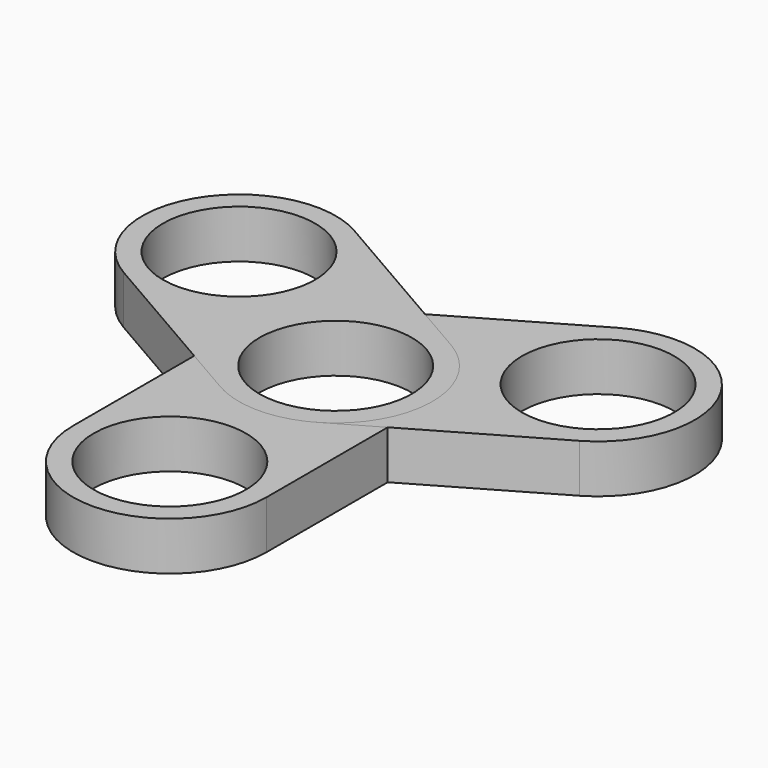
from build123d import *

# Parameters (mm, degrees)
F1_DEPTH        = 177.8
F1_COPIES_COUNT = 3


# Not quite as in the source:
# - a feature of the source that left no trace in its solid (it failed there, or was rolled back) is left out
# - a pattern or mirror of a feature is missing from the dataset's text; its kind, count and spacing are read off the source's solid


with BuildPart() as f1:
    # F0 (on Top) → F1 (new body)
    with BuildSketch(Plane.XY):
        with BuildLine():
            Line((711.2, 0), (635.635, 0))
            ThreePointArc((635.635, 0), (355.6, -280.035), (75.565, 0))
            Line((75.565, 0), (0, 0))
            ThreePointArc((0, 0), (355.6, -355.6), (711.2, 0))
        make_face()
        with BuildLine():
            ThreePointArc((75.565, 0), (355.6, 280.035), (635.635, 0))
            Line((635.635, 0), (711.2, 0))
            ThreePointArc((711.2, 0), (355.6, 355.6), (0, 0))
            Line((0, 0), (75.565, 0))
        make_face()
        with BuildLine():
            ThreePointArc((0, 0), (355.6, 355.6), (711.2, 0))
            Line((711.2, 0), (711.2, 762))
            ThreePointArc((711.2, 762), (355.6, 406.4), (0, 762))
            Line((0, 762), (0, 0))
        make_face()
        with BuildLine():
            Line((635.635, 762), (711.2, 762))
            ThreePointArc((711.2, 762), (355.6, 1117.6), (0, 762))
            Line((0, 762), (75.565, 762))
            ThreePointArc((75.565, 762), (355.6, 1042.035), (635.635, 762))
        make_face()
        with BuildLine():
            ThreePointArc((0, 762), (355.6, 406.4), (711.2, 762))
            Line((711.2, 762), (635.635, 762))
            ThreePointArc((635.635, 762), (355.6, 481.965), (75.565, 762))
            Line((75.565, 762), (0, 762))
        make_face()
    extrude(amount=F1_DEPTH)


with BuildPart() as f1_copies_1:
    # F1_copies: instance of F1
    add(f1.part.rotate(Axis((355.6, 762, 0), (0, 0, 1)), 1 * 360 / F1_COPIES_COUNT))


with BuildPart() as f1_copies_2:
    # F1_copies: instance of F1
    add(f1.part.rotate(Axis((355.6, 762, 0), (0, 0, 1)), 2 * 360 / F1_COPIES_COUNT))


solid = Compound([f1.part, f1_copies_1.part, f1_copies_2.part])
